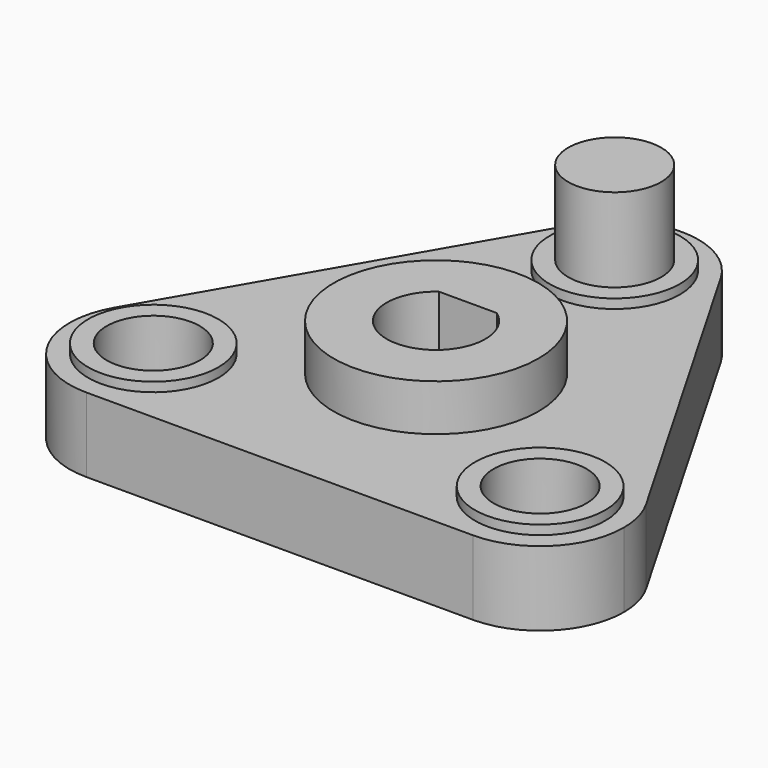
from build123d import *

# Parameters (mm, degrees)
F0_R     = 5.5000004034
F0_R_2   = 2.5
F1_DEPTH = 4
F2_R     = 5.5000004034
F3_DEPTH = 2.5
F4_R     = 3.5
F5_DEPTH = 0.5
F2_R_2   = 3.5
F2_R_3   = 2.5
F6_DEPTH = 0.5
F7_DEPTH = 9


# Not quite as in the source:
# - a feature names something its author has since deleted; it is built from what else it names


with BuildPart() as f1:
    # F0 (on Top) → F1 (new body)
    with BuildSketch(Plane.XY):
        with BuildLine():
            ThreePointArc((-14.2894193359, -3.7500009242), (-9.2276193118, -1.6533344658), (-5.8923048983, -6.0000007153))
            ThreePointArc((-5.8923048983, -6.0000007153), (-7.2103242734, -9.1819811212), (-10.3923045885, -10.5000007153))
            Line((-10.3923045885, -10.5000007153), (10.3923063941, -10.4999992847))
            ThreePointArc((10.3923063941, -10.4999992847), (6.4951930666, -3.7500013262), (14.2894194379, -3.7500019077))
            Line((14.2894194379, -3.7500019077), (3.8971161501, 14.2500004833))
            ThreePointArc((3.8971161501, 14.2500004833), (4.3466679585, 13.1646861286), (4.5000017068, 12.0000004034))
            ThreePointArc((4.5000017068, 12.0000004034), (-1.1646852817, 7.6533330781), (-3.8971148091, 14.2500007515))
            Line((-3.8971148091, 14.2500007515), (-14.2894193359, -3.7500009242))
        make_face()
        Circle(F0_R, mode=Mode.SUBTRACT)
        Circle(F0_R)
        with BuildLine():
            ThreePointArc((1.5576309186, 2.1438950351), (2.3611672891, 1.2030748243), (2.65, 0))
            ThreePointArc((2.65, 0), (-1.2030748243, -2.3611672891), (-1.5576309186, 2.1438950351))
            ThreePointArc((-1.5576309186, 2.1438950351), (0, 2.65), (1.5576309186, 2.1438950351))
        make_face(mode=Mode.SUBTRACT)
        with BuildLine():
            ThreePointArc((3.8971161501, 14.2500004833), (7.479e-07, 16.5000015172), (-3.8971148091, 14.2500007515))
            ThreePointArc((-3.8971148091, 14.2500007515), (-1.1646852817, 7.6533330781), (4.5000017068, 12.0000004034))
            ThreePointArc((4.5000017068, 12.0000004034), (4.3466679585, 13.1646861286), (3.8971161501, 14.2500004833))
        make_face()
        with Locations((5.931e-07, 12.0000004034)):
            Circle(F0_R_2, mode=Mode.SUBTRACT)
        with BuildLine():
            ThreePointArc((-10.3923045885, -10.5000007153), (-7.2103242734, -9.1819811212), (-5.8923048983, -6.0000007153))
            ThreePointArc((-5.8923048983, -6.0000007153), (-9.2276193118, -1.6533344658), (-14.2894193359, -3.7500009242))
            ThreePointArc((-14.2894193359, -3.7500009242), (-14.2894190776, -8.2500009539), (-10.3923045885, -10.5000007153))
        make_face()
        with Locations((-10.3923048983, -6.0000007153)):
            Circle(F0_R_2, mode=Mode.SUBTRACT)
        with BuildLine():
            ThreePointArc((14.2894194379, -3.7500019077), (6.4951930666, -3.7500013262), (10.3923063941, -10.4999992847))
            ThreePointArc((10.3923063941, -10.4999992847), (13.5742856976, -9.1819801095), (14.8923046537, -6.0000007153))
            ThreePointArc((14.8923046537, -6.0000007153), (14.7389709921, -4.8353156487), (14.2894194379, -3.7500019077))
        make_face()
        with Locations((10.3923060844, -6.0000007153)):
            Circle(F0_R_2, mode=Mode.SUBTRACT)
        with BuildLine():
            Line((-1.5576309186, 2.1438950351), (1.5576309186, 2.1438950351))
            ThreePointArc((1.5576309186, 2.1438950351), (0, 2.65), (-1.5576309186, 2.1438950351))
        make_face()
    extrude(amount=F1_DEPTH)

    # F2 (on face) → F3 (join)
    with BuildSketch(Plane.XY.offset(4)):
        Circle(F2_R)
        with BuildLine():
            ThreePointArc((1.5576309186, 2.1438950351), (0, -2.65), (-1.5576309186, 2.1438950351))
            Line((-1.5576309186, 2.1438950351), (1.5576309186, 2.1438950351))
        make_face(mode=Mode.SUBTRACT)
    extrude(amount=F3_DEPTH)

    # F2 (on face) → F6 (join)
    with BuildSketch(Plane.XY.offset(4)):
        with Locations((5.931e-07, 12.0000004034)):
            Circle(F2_R_2)
        with Locations((5.931e-07, 12.0000004034)):
            Circle(F2_R_3, mode=Mode.SUBTRACT)
        with Locations((-10.3923048983, -6.0000007153)):
            Circle(F2_R_2)
        with Locations((-10.3923048983, -6.0000007153)):
            Circle(F2_R_3, mode=Mode.SUBTRACT)
        with Locations((10.3923060844, -6.0000007153)):
            Circle(F2_R_2)
        with Locations((10.3923060844, -6.0000007153)):
            Circle(F2_R_3, mode=Mode.SUBTRACT)
    extrude(amount=F6_DEPTH)


with BuildPart() as f5:
    # F4 (on face) → F5 (new body)
    with BuildSketch(Plane(origin=(0, 0, 0), x_dir=(1, 0, 0), z_dir=(0, 0, -1))):
        Circle(F4_R)
        with BuildLine():
            ThreePointArc((-1.5576309186, -2.1438950351), (-1.2030748243, 2.3611672891), (2.65, 0))
            ThreePointArc((2.65, 0), (2.3611672891, -1.2030748243), (1.5576309186, -2.1438950351))
            ThreePointArc((1.5576309186, -2.1438950351), (0, -2.65), (-1.5576309186, -2.1438950351))
        make_face(mode=Mode.SUBTRACT)
    extrude(amount=F5_DEPTH)


with BuildPart() as f7:
    # F0 (on Top) → F7 (new body)
    with BuildSketch(Plane.XY):
        with Locations((5.931e-07, 12.0000004034)):
            Circle(F0_R_2)
    extrude(amount=F7_DEPTH)


solid = Compound([f1.part, f5.part, f7.part])
